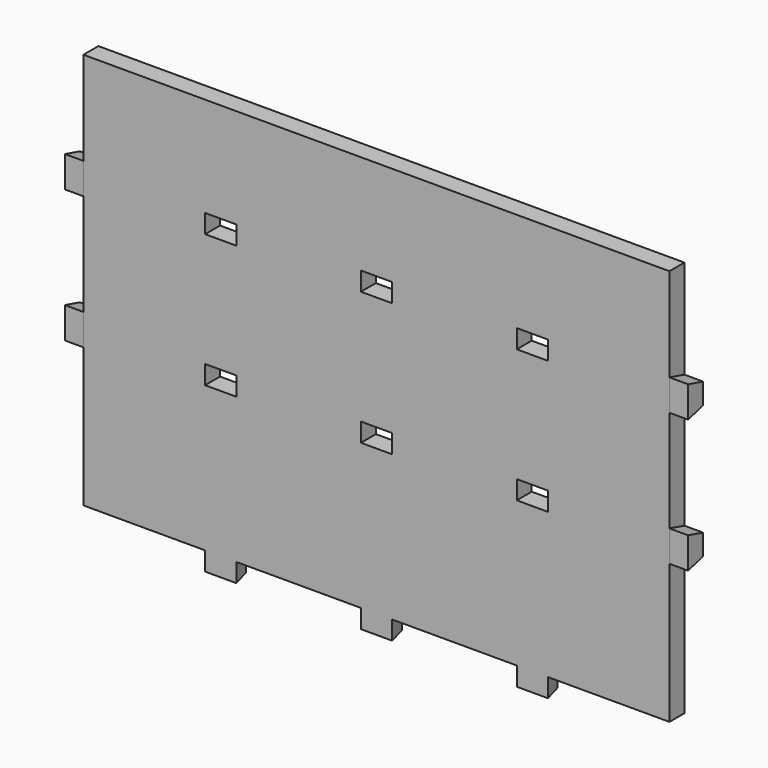
from build123d import *

# Parameters (mm, degrees)
F4_W      = 564.1347765923
F4_H      = 381.999976933
F5_DEPTH  = 18
F6_DEPTH  = 17.9999992251
F7_DEPTH  = 18.0000689332
F10_DEPTH = 17.8651544745
F12_DEPTH = 25


with BuildPart() as f5:
    # F4 (on plane+point) → F5 (new body)
    with BuildSketch(Plane.XZ.offset(-129.0130399809)):
        with Locations((-0.1316666603, 208.9999876916)):
            Rectangle(F4_W, F4_H)
    extrude(amount=F5_DEPTH)

    # F0 (on Top) → F6 (join, through all)
    with BuildSketch(Plane.XY):
        Polygon((149.935790569, 129.0130399809), (139.935790569, 129.0130399809), (134.935790569, 111.0130399809), (164.935790569, 111.0130399809), (159.935790569, 129.0130399809), align=None)
        Polygon((-0.064209431, 129.0130399809), (-10.064209431, 129.0130399809), (-15.064209431, 111.0130399809), (-0.064209431, 111.0130399809), (14.935790569, 111.0130399809), (9.935790569, 129.0130399809), align=None)
        Polygon((-150.064209431, 129.0130399809), (-160.064209431, 129.0130399809), (-165.064209431, 111.0130399809), (-135.064209431, 111.0130399809), (-140.064209431, 129.0130399809), align=None)
    extrude(amount=F6_DEPTH)

    # F3 (on plane+point) → F7 (join, through all)
    with BuildSketch(Plane.YZ.offset(299.935790569)):
        Polygon((111.0131509304, 152), (129.0131509304, 157), (129.0131509304, 177), (111.0131509304, 182), align=None)
        Polygon((129.0131509304, 295), (129.0131509304, 305), (111.0131509304, 310), (111.0131509304, 295), (111.0131509304, 280), (129.0131509304, 285), align=None)
    extrude(amount=-F7_DEPTH)

    # F9 (on offset) → F10 (join, through all)
    with BuildSketch(Plane.YZ.offset(-300.064209431)):
        Polygon((129.0131062269, 295), (129.0131062269, 305), (111.0131062269, 310), (111.0131062269, 295), (111.0131062269, 280), (129.0131062269, 285), align=None)
        Polygon((111.0131062269, 152), (129.0131062269, 157), (129.0131062269, 177), (111.0131062269, 182), align=None)
    extrude(amount=F10_DEPTH)

    # F11 (on plane+point) → F12 (cut)
    with BuildSketch(Plane.XZ.offset(-129.0130399809)):
        Polygon((164.9357974529, 167), (164.9357974529, 175.9999990463), (149.935790569, 175.9999990463), (134.9357962608, 175.9999990463), (134.9357962608, 167), (134.9357962608, 158.0000072718), (149.935790569, 158.0000072718), (164.9357974529, 158.0000072718), align=None)
        Polygon((149.935790569, 286.0000133514), (164.9357974529, 286.0000133514), (164.9357974529, 295), (164.9357974529, 303.9999902248), (149.935790569, 303.9999902248), (134.9357962608, 303.9999902248), (134.9357962608, 295), (134.9357962608, 286.0000133514), align=None)
        Polygon((14.9357905611, 167), (14.9357905611, 175.9999990463), (-15.0642096996, 175.9999990463), (-15.0642096996, 167), (-15.0642096996, 158.0000072718), (14.9357905611, 158.0000072718), align=None)
        Polygon((-15.0642096996, 286.0000133514), (14.9357905611, 286.0000133514), (14.9357905611, 295), (14.9357905611, 303.9999902248), (-15.0642096996, 303.9999902248), (-15.0642096996, 295), align=None)
        Polygon((-135.064214468, 167), (-135.064214468, 175.9999990463), (-165.0642156601, 175.9999990463), (-165.0642156601, 167), (-165.0642156601, 158.0000072718), (-135.064214468, 158.0000072718), align=None)
        Polygon((-165.0642156601, 286.0000133514), (-135.064214468, 286.0000133514), (-135.064214468, 295), (-135.064214468, 303.9999902248), (-165.0642156601, 303.9999902248), (-165.0642156601, 295), align=None)
    extrude(amount=F12_DEPTH, mode=Mode.SUBTRACT)


solid = f5.part
